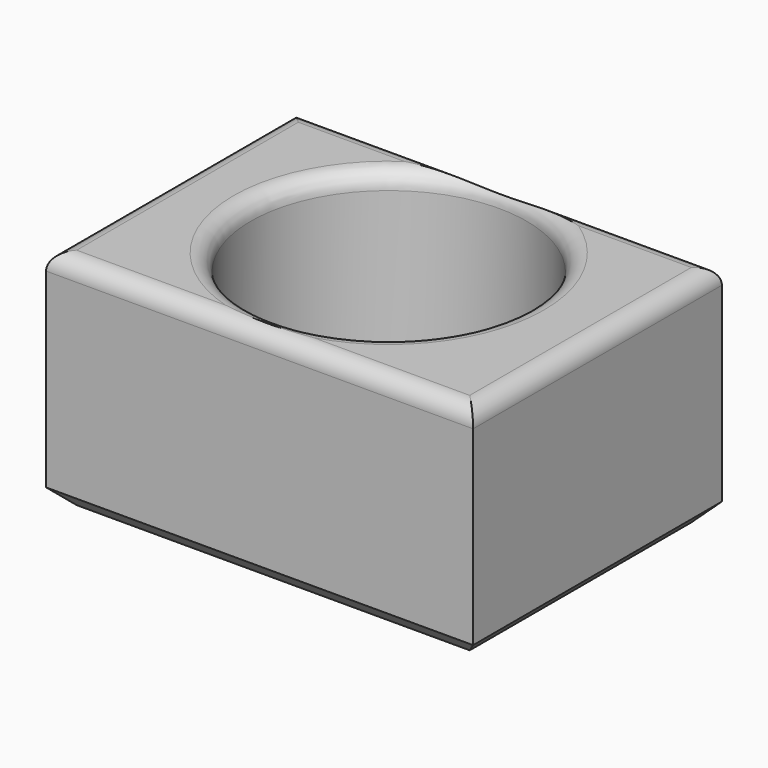
from build123d import *

# Parameters (mm, degrees)
F0_W        = 125.5629397929
F0_H        = 91.4415977895
F0_R        = 40.6040371895
F1_DEPTH    = 60
F2_W        = 118.2770989835
F2_H        = 87.5040702522
F3_DEPTH    = 6
F4_T1_DEPTH = 150.5629397929
F4_T3_DEPTH = 116.4415977895
F5_SIZE     = 5


# Not quite as in the source:
# - a fillet or chamfer that OpenCascade refuses, or shapes differently, is made with other operations: its cross-section is extruded or revolved along the edge and cut away or added


with BuildPart() as f1:
    # F0 (on Top) → F1 (new body)
    with BuildSketch(Plane.XY):
        with Locations((1.0034125298, -8.6029302329)):
            Rectangle(F0_W, F0_H)
        with Locations((0, -5.6129307486)):
            Circle(F0_R, mode=Mode.SUBTRACT)
    extrude(amount=F1_DEPTH)

    # F2 (on face) → F3 (join)
    with BuildSketch(Plane(origin=(0, 0, 0), x_dir=(1, 0, 0), z_dir=(0, 0, -1))):
        Polygon((63.7848824263, -37.1178686619), (63.7848824263, 54.3237291276), (-61.7780573666, 54.3237291276), (-61.7780573666, -37.1178686619), (-58.5906021297, -37.1178686619), (-58.5906021297, 50.3862015903), (59.6864968538, 50.3862015903), (59.6864968538, -37.1178686619), align=None)
        with Locations((0.5479473621, 6.6341664642)):
            Rectangle(F2_W, F2_H)
    extrude(amount=F3_DEPTH)

    # F4: fillet of radius 5 on 5 edges, made by hand

    # F4_s2 → F4_t1 (cut)
    with BuildSketch(Plane.YZ.offset(-74.2780573666)):
        with BuildLine():
            ThreePointArc((37.1178686619, 55), (35.6534025678, 58.5355339059), (32.1178686619, 60))
            Line((32.1178686619, 60), (37.1178686619, 60))
            Line((37.1178686619, 60), (37.1178686619, 55))
        make_face()
        with BuildLine():
            ThreePointArc((-49.3237291276, 60), (-52.8592630336, 58.5355339059), (-54.3237291276, 55))
            Line((-54.3237291276, 55), (-54.3237291276, 60))
            Line((-54.3237291276, 60), (-49.3237291276, 60))
        make_face()
    extrude(amount=F4_T1_DEPTH, mode=Mode.SUBTRACT)

    # F4_s4 → F4_t3 (cut)
    with BuildSketch(Plane.XZ.offset(-49.6178686619)):
        with BuildLine():
            ThreePointArc((63.7848824263, 55), (62.3204163322, 58.5355339059), (58.7848824263, 60))
            Line((58.7848824263, 60), (63.7848824263, 60))
            Line((63.7848824263, 60), (63.7848824263, 55))
        make_face()
        with BuildLine():
            ThreePointArc((-61.7780573666, 55), (-60.3135912725, 58.5355339059), (-56.7780573666, 60))
            Line((-56.7780573666, 60), (-61.7780573666, 60))
            Line((-61.7780573666, 60), (-61.7780573666, 55))
        make_face()
    extrude(amount=F4_T3_DEPTH, mode=Mode.SUBTRACT)

    # F4_s5 → F4_t6 (revolve, cut)
    with BuildSketch(Plane.XZ.offset(5.6129307486)):
        with BuildLine():
            ThreePointArc((45.6040371895, 60), (42.0685032836, 58.5355339059), (40.6040371895, 55))
            Line((40.6040371895, 55), (40.6040371895, 60))
            Line((40.6040371895, 60), (45.6040371895, 60))
        make_face()
    revolve(axis=Axis((0, -5.6129307486, 60), (0, 0, 1)), mode=Mode.SUBTRACT)

    # F5
    f5_edges = [f1.edges().sort_by_distance(p)[0] for p in [
        (1.003413, 37.117869, -6),
        (63.784882, -8.60293, -6),
        (1.003413, -54.323729, -6),
        (-61.778057, -8.60293, -6),
    ]]
    chamfer(f5_edges, length=F5_SIZE)


solid = f1.part
